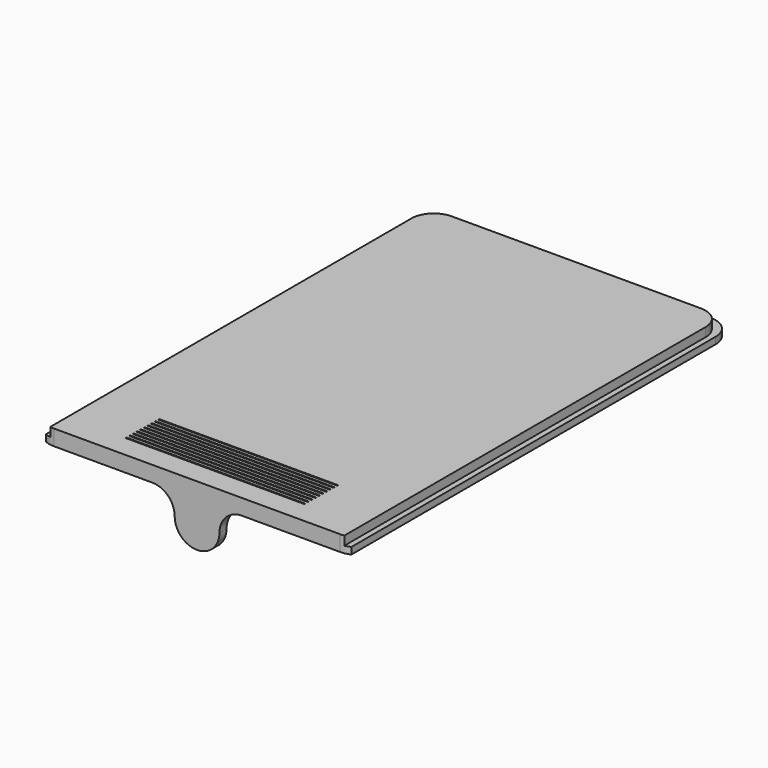
from build123d import *

# Parameters (mm, degrees)
F1_DEPTH  = 106
F2_W      = 68.25
F2_H      = 1.5
F3_DEPTH  = 1.25
F4_R      = 5
F6_DEPTH  = 25
F7_W      = 10
F7_H      = 10
F8_DEPTH  = 2
F9_R      = 4.99999
F10_W     = 5
F10_H     = 5
F11_DEPTH = 1
F12_W     = 40
F12_H     = 0.25
F13_DEPTH = 1


# Not quite as in the source:
# - a fillet or chamfer is up to 0.001 mm smaller than in the source, because OpenCascade refuses the exact size


with BuildPart() as f1:
    # F0 (on Front) → F1 (new body)
    with BuildSketch(Plane.XZ):
        Polygon((32.875, 1.5), (32.875, 3.5), (-32.875, 3.5), (-32.875, 1.5), (-34.125, 1.5), (-34.125, 0), (34.125, 0), (34.125, 1.5), align=None)
    extrude(amount=-F1_DEPTH)

    # F2 (on face) → F3 (join)
    with BuildSketch(Plane(origin=(0, 106, 0), x_dir=(-1, 0, 0), z_dir=(0, 1, 0))):
        with Locations((0, 0.75)):
            Rectangle(F2_W, F2_H)
    extrude(amount=F3_DEPTH)

    # F4
    f4_edges = [f1.edges().sort_by_distance(p)[0] for p in [
        (34.125, 107.25, 0.75),
        (-34.125, 107.25, 0.75),
        (-32.875, 106, 2.5),
        (32.875, 106, 2.5),
    ]]
    fillet(f4_edges, radius=F4_R)

    # F5 (on Top) → F6 (cut)
    with BuildSketch(Plane.XY):
        with BuildLine():
            ThreePointArc((-32, 0), (-35.5355339059, 1.4644660941), (-37, 5))
            Line((-37, 5), (-47.4459486902, 5.1317643374))
            Line((-47.4459486902, 5.1317643374), (-32.4784885049, -8.2395952195))
            Line((-32.4784885049, -8.2395952195), (-32, 0))
        make_face()
        with BuildLine():
            Line((47.8749121428, 4.8458835855), (37, 4.9999998882))
            ThreePointArc((37, 4.9999998882), (35.5355339059, 1.4644659823), (32, -1.118e-07))
            Line((32, -1.118e-07), (31.699370116, -9.054190591))
            Line((31.699370116, -9.054190591), (47.8749121428, 4.8458835855))
        make_face()
    extrude(amount=F6_DEPTH, mode=Mode.SUBTRACT)

    # F7 (on face) → F8 (join)
    with BuildSketch(Plane.XZ):
        with Locations((0, -5)):
            Rectangle(F7_W, F7_H)
    extrude(amount=-F8_DEPTH)

    # F9 (radius 5 in the source; OpenCascade refuses exactly that, so slightly less here)
    f9_edges = [f1.edges().sort_by_distance(p)[0] for p in [
        (5, 1, 0),
        (-5, 1, 0),
        (-5, 1, -10),
        (5, 1, -10),
    ]]
    fillet(f9_edges, radius=F9_R)

    # F10 (on face) → F11 (cut)
    with BuildSketch(Plane(origin=(0, 2, 0), x_dir=(-1, 0, 0), z_dir=(0, 1, 0))):
        with Locations((0, -2.5)):
            Rectangle(F10_W, F10_H)
    extrude(amount=-F11_DEPTH, mode=Mode.SUBTRACT)

    # F12 (on face) → F13 (cut)
    with BuildSketch(Plane.XY.offset(3.5)):
        with Locations((0, 5.125)):
            Rectangle(F12_W, F12_H)
        with Locations((0.0169467185, 6.1248563941)):
            Rectangle(F12_W, F12_H)
        with Locations((0.0338934371, 7.1247127881)):
            Rectangle(F12_W, F12_H)
        with Locations((0.0508401556, 8.1245691822)):
            Rectangle(F12_W, F12_H)
        with Locations((0.0677868742, 9.1244255762)):
            Rectangle(F12_W, F12_H)
        with Locations((0.0847335927, 10.1242819703)):
            Rectangle(F12_W, F12_H)
        with Locations((0.1016803113, 11.1241383643)):
            Rectangle(F12_W, F12_H)
        with Locations((0.1186270298, 12.1239947584)):
            Rectangle(F12_W, F12_H)
        with Locations((0.1355737483, 13.1238511524)):
            Rectangle(F12_W, F12_H)
        with Locations((0.1525204669, 14.1237075465)):
            Rectangle(F12_W, F12_H)
    extrude(amount=-F13_DEPTH, mode=Mode.SUBTRACT)


solid = f1.part
